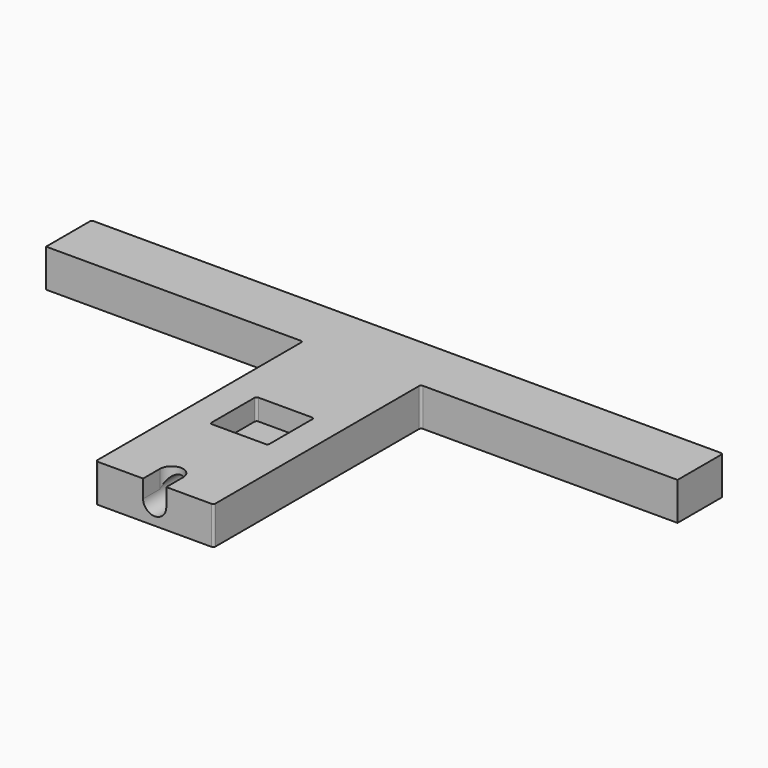
from build123d import *

# Parameters (mm, degrees)
F1_DEPTH = 3.6
F2_R     = 1.1
F3_DEPTH = 8
F4_W     = 2.2
F4_H     = 2
F5_DEPTH = 1.7
F6_R     = 1.6
F7_DEPTH = 1.2
F8_W     = 5.5
F8_H     = 5.5
F9_DEPTH = 2
F10_R    = 0.2


# Not quite as in the source:
# - a feature names something its author has since deleted; it is built from what else it names


with BuildPart() as f1:
    # F0 (on Top) → F1 (new body)
    with BuildSketch(Plane.XY):
        Polygon((30, 15), (-30, 15), (-30, 9.6), (-5.6, 9.6), (-5.6, -15), (5.6, -15), (5.6, 9.6), (30, 9.6), align=None)
    extrude(amount=F1_DEPTH)

    # F2 (on face) → F3 (cut)
    with BuildSketch(Plane.XZ.offset(15)):
        with Locations((0, 1.9)):
            Circle(F2_R)
    extrude(amount=-F3_DEPTH, mode=Mode.SUBTRACT)

    # F4 (on face) → F5 (cut)
    with BuildSketch(Plane.XY.offset(3.6)):
        with Locations((0, -14)):
            Rectangle(F4_W, F4_H)
        with BuildLine():
            ThreePointArc((1.1, -13), (0, -11.9), (-1.1, -13))
            Line((-1.1, -13), (1.1, -13))
        make_face()
    extrude(amount=-F5_DEPTH, mode=Mode.SUBTRACT)

    # F6 (on face) → F7 (cut)
    with BuildSketch(Plane(origin=(0, 0, 0), x_dir=(1, 0, 0), z_dir=(0, 0, -1))):
        with Locations((0, 5)):
            Circle(F6_R)
        with Locations((0, -3.3)):
            Circle(F6_R)
        with Locations((25, -12.3)):
            Circle(F6_R)
        with Locations((-25, -12.3)):
            Circle(F6_R)
        with Locations((0, -12.3)):
            Circle(F6_R)
    extrude(amount=-F7_DEPTH, mode=Mode.SUBTRACT)

    # F8 (on face) → F9 (cut)
    with BuildSketch(Plane.XY.offset(3.6)):
        with Locations((0, -2.25)):
            Rectangle(F8_W, F8_H)
    extrude(amount=-F9_DEPTH, mode=Mode.SUBTRACT)

    # F10
    f10_edges = [f1.edges().sort_by_distance(p)[0] for p in [
        (-5.6, 9.6, 1.8),
        (5.6, 9.6, 1.8),
        (30, 15, 1.8),
        (-30, 15, 1.8),
        (-2.75, 0.5, 2.6),
        (2.75, 0.5, 2.6),
        (2.75, -5, 2.6),
        (-2.75, -5, 2.6),
        (5.6, -15, 1.8),
        (-5.6, -15, 1.8),
    ]]
    fillet(f10_edges, radius=F10_R)


solid = f1.part
